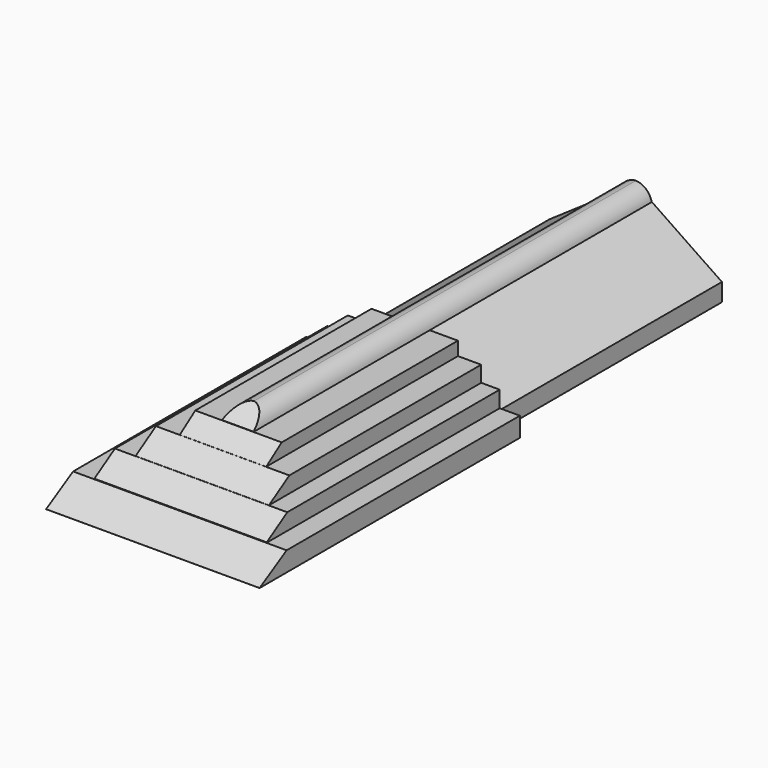
from build123d import *

# Parameters (mm, degrees)
F0_W         = 192.698314786
F0_H         = 17.6181327552
F1_DEPTH     = 293.624
F2_SIZE2     = 17.5976362049
F2_SIZE      = 30.48
F3_W         = 155.5479988456
F3_H         = 14.7782256827
F4_DEPTH     = 262.8138
F5_SIZE2     = 23.1696433115
F5_SIZE      = 14.478
F6_W         = 120.3552596271
F6_H         = 14.3881891854
F7_DEPTH     = 239.5982
F8_T4_DEPTH  = 240.1584395307
F9_W         = 77.968429774
F9_H         = 12.2494040988
F10_DEPTH    = 216.408
F11_T4_DEPTH = 168.8399476849
F12_W        = 28.5819442943
F12_H        = 12.4438395724
F13_DEPTH    = 198.628
F14_SIZE2    = 18.2636685711
F14_SIZE     = 12.319
F15_T1_DEPTH = 255.6446994283
F17_DEPTH    = 250.698
F18_DEPTH    = 250.444


# Not quite as in the source:
# - a fillet or chamfer that OpenCascade refuses, or shapes differently, is made with other operations: its cross-section is extruded or revolved along the edge and cut away or added


with BuildPart() as f1:
    # F0 (on Front) → F1 (new body)
    with BuildSketch(Plane.XZ):
        with Locations((2.8250664473, -34.9617386237)):
            Rectangle(F0_W, F0_H)
    extrude(amount=F1_DEPTH)

    # F2
    f2_edges = [f1.edges().sort_by_distance(p)[0] for p in [
        (2.825066, -293.624, -26.152672),
    ]]
    f2_side = f1.faces().sort_by_distance((2.825066, -146.812, -26.152672))[0]
    chamfer(f2_edges, length=F2_SIZE, length2=F2_SIZE2, reference=f2_side)

    # F3 (on face) → F4 (join)
    with BuildSketch(Plane(origin=(0, 0, 0), x_dir=(-1, 0, 0), z_dir=(0, 1, 0))):
        with Locations((-3.2139383256, -18.7635594048)):
            Rectangle(F3_W, F3_H)
    extrude(amount=-F4_DEPTH)

    # F5
    f5_edges = [f1.edges().sort_by_distance(p)[0] for p in [
        (3.213938, -262.8138, -11.374447),
    ]]
    f5_side = f1.faces().sort_by_distance((3.213938, -262.8138, -18.763559))[0]
    chamfer(f5_edges, length=F5_SIZE, length2=F5_SIZE2, reference=f5_side)

    # F6 (on face) → F7 (join)
    with BuildSketch(Plane(origin=(0, 0, 0), x_dir=(-1, 0, 0), z_dir=(0, 1, 0))):
        with Locations((-4.0888953954, -4.1803519707)):
            Rectangle(F6_W, F6_H)
    extrude(amount=-F7_DEPTH)

    # F8: chamfer of 14.478 x 23.1696433115 on 1 edges, made by hand


with BuildPart() as f8_tool2:
    # F8_s3 → F8_t4 (new body)
    with BuildSketch(Plane.YZ.offset(-115.99032437)):
        Polygon((-239.5982, -11.464257378), (-216.4285566885, 3.013742622), (-239.5982, 3.013742622), align=None)
    extrude(amount=F8_T4_DEPTH)

    split(bisect_by=Plane.XY.offset(-11.3744465634), keep=Keep.TOP)


with BuildPart() as f1_1:
    add(f1.part)

    # F8_t1: cut F8_tool2
    add(f8_tool2.part, mode=Mode.SUBTRACT)

    # F9 (on face) → F10 (join)
    with BuildSketch(Plane(origin=(0, 0, 0), x_dir=(-1, 0, 0), z_dir=(0, 1, 0))):
        with Locations((-4.2833294719, 9.1384446714)):
            Rectangle(F9_W, F9_H)
    extrude(amount=-F10_DEPTH)

    # F11: chamfer of 12.319 x 17.5933552951 on 1 edges, made by hand


with BuildPart() as f11_tool2:
    # F11_s3 → F11_t4 (new body)
    with BuildSketch(Plane.YZ.offset(-80.1366443705)):
        Polygon((-216.408, 2.9441467208), (-198.8146447049, 15.2631467208), (-216.408, 15.2631467208), align=None)
    extrude(amount=F11_T4_DEPTH)

    split(bisect_by=Plane.XY.offset(3.013742622), keep=Keep.TOP)


with BuildPart() as f1_2:
    add(f1_1.part)

    # F11_t1: cut F11_tool2
    add(f11_tool2.part, mode=Mode.SUBTRACT)

    # F12 (on face) → F13 (join)
    with BuildSketch(Plane(origin=(0, 0, 0), x_dir=(-1, 0, 0), z_dir=(0, 1, 0))):
        with Locations((-3.5055889748, 21.485066507)):
            Rectangle(F12_W, F12_H)
    extrude(amount=-F13_DEPTH)

    # F14
    f14_edges = [f1_2.edges().sort_by_distance(p)[0] for p in [
        (3.505589, -198.628, 27.706986),
    ]]
    f14_side = f1_2.faces().sort_by_distance((3.505589, -198.628, 21.485067))[0]
    chamfer(f14_edges, length=F14_SIZE, length2=F14_SIZE2, reference=f14_side)

    # F15: fillet of radius 15.3302561211 on 2 edges, made by hand

    # F15_s2 → F15_t1 (cut)
    with BuildSketch(Plane.XZ.offset(-37.6401839997)):
        with BuildLine():
            ThreePointArc((2.7404875221, 27.7069862932), (12.5069415299, 24.1933764328), (17.7965611219, 15.2631467208))
            Line((17.7965611219, 15.2631467208), (17.7965611219, 27.7069862932))
            Line((17.7965611219, 27.7069862932), (2.7404875221, 27.7069862932))
        make_face()
        with BuildLine():
            ThreePointArc((-10.7853831723, 15.2631467208), (-5.4957635803, 24.1933764328), (4.2706904276, 27.7069862932))
            Line((4.2706904276, 27.7069862932), (-10.7853831723, 27.7069862932))
            Line((-10.7853831723, 27.7069862932), (-10.7853831723, 15.2631467208))
        make_face()
    extrude(amount=F15_T1_DEPTH, mode=Mode.SUBTRACT)

    # F16 (on face) → F17 (join)
    with BuildSketch(Plane(origin=(0, 0, 0), x_dir=(-1, 0, 0), z_dir=(0, 1, 0))):
        Polygon((-80.9879377484, -27.7069862932), (-80.9879377484, -43.7708050013), (74.5600610971, -43.7708050013), (74.5600610971, -28.4847263247), (10.7853831723, 15.2631467208), (-17.7965611219, 15.2631467208), align=None)
    extrude(amount=F17_DEPTH)

    # F18 (add): a face of the model
    f18_faces = [f1_2.faces().sort_by_distance(p)[0] for p in [
        (3.5055889748, 0, 20.394937783),
    ]]
    extrude(f18_faces, amount=F18_DEPTH)


solid = f1_2.part
